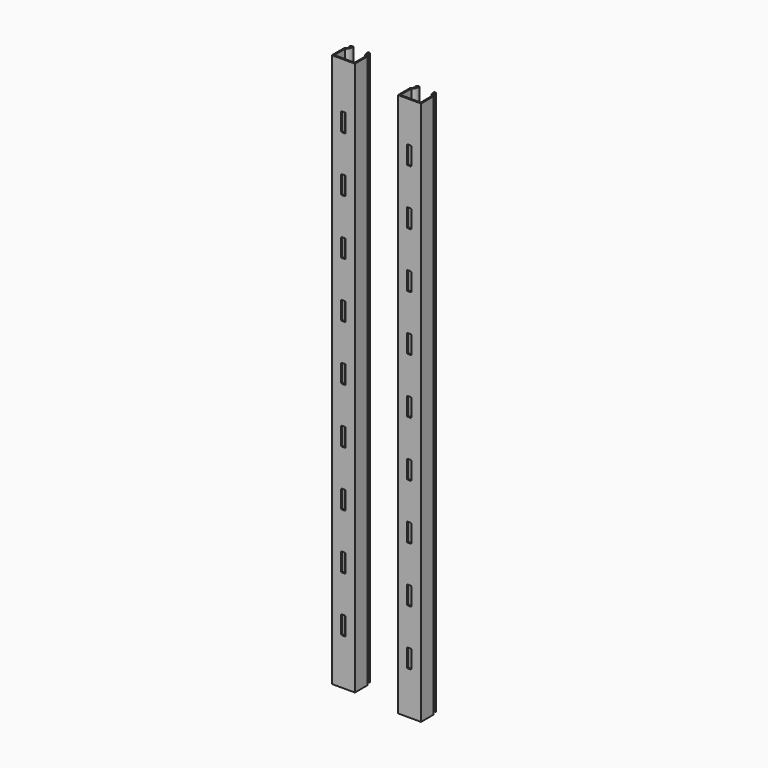
from build123d import *

# Parameters (mm, degrees)
F1_DEPTH = 300
F3_DEPTH = 25
F5_DEPTH = 295
F7_DEPTH = 25


# Not quite as in the source:
# - a feature names something its author has since deleted; it is built from what else it names


with BuildPart() as f1:
    # F0 (on Top) → F1 (new body, symmetric)
    with BuildSketch(Plane.XY):
        with BuildLine():
            Line((-95.8714708686, 0), (-70.8714708686, 0))
            Line((-70.8714708686, 0), (-70.8714708686, 17))
            ThreePointArc((-70.8714708686, 17), (-73.0196975842, 19.1110639706), (-73.8714708686, 22))
            Line((-73.8714708686, 22), (-72.3714708686, 22))
            ThreePointArc((-72.3714708686, 22), (-73.4661714465, 23.4241895875), (-75.2608686682, 23.5))
            ThreePointArc((-75.2608686682, 23.5), (-74.8489206928, 19.4392699226), (-72.3714708686, 16.1955880232))
            Line((-72.3714708686, 16.1955880232), (-72.3714708686, 1.5))
            Line((-72.3714708686, 1.5), (-83.3714708686, 1.5))
            Line((-83.3714708686, 1.5), (-94.3714708686, 1.5))
            Line((-94.3714708686, 1.5), (-94.3714708686, 16.1955880232))
            ThreePointArc((-94.3714708686, 16.1955880232), (-91.8940210443, 19.4392699226), (-91.482073069, 23.5))
            ThreePointArc((-91.482073069, 23.5), (-93.2767702907, 23.4241895875), (-94.3714708686, 22))
            Line((-94.3714708686, 22), (-92.8714708686, 22))
            ThreePointArc((-92.8714708686, 22), (-93.723244153, 19.1110639706), (-95.8714708686, 17))
            Line((-95.8714708686, 17), (-95.8714708686, 0))
        make_face()
    extrude(amount=F1_DEPTH, both=True)

    # F2 (on face) → F3 (cut)
    with BuildSketch(Plane.XZ):
        with BuildLine():
            Line((-84.8714708686, -10), (-83.3714708686, -10))
            Line((-83.3714708686, -10), (-83.3714708686, 0))
            Line((-83.3714708686, 0), (-83.3714708686, 10))
            Line((-83.3714708686, 10), (-84.8714708686, 10))
            ThreePointArc((-84.8714708686, 10), (-85.5785776498, 9.7071067812), (-85.8714708686, 9))
            Line((-85.8714708686, 9), (-85.8714708686, -9))
            ThreePointArc((-85.8714708686, -9), (-85.5785776498, -9.7071067812), (-84.8714708686, -10))
        make_face()
        with BuildLine():
            Line((-83.3714708686, 10), (-83.3714708686, 0))
            Line((-83.3714708686, 0), (-80.8714708686, 0))
            Line((-80.8714708686, 0), (-80.8714708686, 9))
            ThreePointArc((-80.8714708686, 9), (-81.1643640874, 9.7071067812), (-81.8714708686, 10))
            Line((-81.8714708686, 10), (-83.3714708686, 10))
        make_face()
        with BuildLine():
            Line((-83.3714708686, 0), (-83.3714708686, -10))
            Line((-83.3714708686, -10), (-81.8714708686, -10))
            ThreePointArc((-81.8714708686, -10), (-81.1643640874, -9.7071067812), (-80.8714708686, -9))
            Line((-80.8714708686, -9), (-80.8714708686, 0))
            Line((-80.8714708686, 0), (-83.3714708686, 0))
        make_face()
        with BuildLine():
            Line((-81.8714708686, -50), (-83.3714708686, -50))
            Line((-83.3714708686, -50), (-83.3714708686, -60))
            Line((-83.3714708686, -60), (-80.8714708686, -60))
            Line((-80.8714708686, -60), (-80.8714708686, -51))
            ThreePointArc((-80.8714708686, -51), (-81.1643640874, -50.2928932188), (-81.8714708686, -50))
        make_face()
        with BuildLine():
            Line((-80.8714708686, -60), (-83.3714708686, -60))
            Line((-83.3714708686, -60), (-83.3714708686, -70))
            Line((-83.3714708686, -70), (-81.8714708686, -70))
            ThreePointArc((-81.8714708686, -70), (-81.1643640874, -69.7071067812), (-80.8714708686, -69))
            Line((-80.8714708686, -69), (-80.8714708686, -60))
        make_face()
        with BuildLine():
            Line((-83.3714708686, -60), (-83.3714708686, -50))
            Line((-83.3714708686, -50), (-84.8714708686, -50))
            ThreePointArc((-84.8714708686, -50), (-85.5785776498, -50.2928932188), (-85.8714708686, -51))
            Line((-85.8714708686, -51), (-85.8714708686, -60))
            Line((-85.8714708686, -60), (-83.3714708686, -60))
        make_face()
        with BuildLine():
            Line((-83.3714708686, -70), (-83.3714708686, -60))
            Line((-83.3714708686, -60), (-85.8714708686, -60))
            Line((-85.8714708686, -60), (-85.8714708686, -69))
            ThreePointArc((-85.8714708686, -69), (-85.5785776498, -69.7071067812), (-84.8714708686, -70))
            Line((-84.8714708686, -70), (-83.3714708686, -70))
        make_face()
        with BuildLine():
            Line((-81.8714708686, -110), (-83.3714708686, -110))
            Line((-83.3714708686, -110), (-83.3714708686, -120))
            Line((-83.3714708686, -120), (-80.8714708686, -120))
            Line((-80.8714708686, -120), (-80.8714708686, -111))
            ThreePointArc((-80.8714708686, -111), (-81.1643640874, -110.2928932188), (-81.8714708686, -110))
        make_face()
        with BuildLine():
            Line((-80.8714708686, -120), (-83.3714708686, -120))
            Line((-83.3714708686, -120), (-83.3714708686, -130))
            Line((-83.3714708686, -130), (-81.8714708686, -130))
            ThreePointArc((-81.8714708686, -130), (-81.1643640874, -129.7071067812), (-80.8714708686, -129))
            Line((-80.8714708686, -129), (-80.8714708686, -120))
        make_face()
        with BuildLine():
            Line((-83.3714708686, -120), (-83.3714708686, -110))
            Line((-83.3714708686, -110), (-84.8714708686, -110))
            ThreePointArc((-84.8714708686, -110), (-85.5785776498, -110.2928932188), (-85.8714708686, -111))
            Line((-85.8714708686, -111), (-85.8714708686, -129))
            ThreePointArc((-85.8714708686, -129), (-85.5785776498, -129.7071067812), (-84.8714708686, -130))
            Line((-84.8714708686, -130), (-83.3714708686, -130))
            Line((-83.3714708686, -130), (-83.3714708686, -120))
        make_face()
        with BuildLine():
            Line((-83.3714708686, -180), (-83.3714708686, -170))
            Line((-83.3714708686, -170), (-84.8714708686, -170))
            ThreePointArc((-84.8714708686, -170), (-85.5785776498, -170.2928932188), (-85.8714708686, -171))
            Line((-85.8714708686, -171), (-85.8714708686, -180))
            Line((-85.8714708686, -180), (-83.3714708686, -180))
        make_face()
        with BuildLine():
            Line((-83.3714708686, -190), (-83.3714708686, -180))
            Line((-83.3714708686, -180), (-85.8714708686, -180))
            Line((-85.8714708686, -180), (-85.8714708686, -189))
            ThreePointArc((-85.8714708686, -189), (-85.5785776498, -189.7071067812), (-84.8714708686, -190))
            Line((-84.8714708686, -190), (-83.3714708686, -190))
        make_face()
        with BuildLine():
            Line((-80.8714708686, -189), (-80.8714708686, -180))
            Line((-80.8714708686, -180), (-83.3714708686, -180))
            Line((-83.3714708686, -180), (-83.3714708686, -190))
            Line((-83.3714708686, -190), (-81.8714708686, -190))
            ThreePointArc((-81.8714708686, -190), (-81.1643640874, -189.7071067812), (-80.8714708686, -189))
        make_face()
        with BuildLine():
            Line((-81.8714708686, -170), (-83.3714708686, -170))
            Line((-83.3714708686, -170), (-83.3714708686, -180))
            Line((-83.3714708686, -180), (-80.8714708686, -180))
            Line((-80.8714708686, -180), (-80.8714708686, -171))
            ThreePointArc((-80.8714708686, -171), (-81.1643640874, -170.2928932188), (-81.8714708686, -170))
        make_face()
        with BuildLine():
            Line((-83.3714708686, -250), (-83.3714708686, -240))
            Line((-83.3714708686, -240), (-83.3714708686, -230))
            Line((-83.3714708686, -230), (-84.8714708686, -230))
            ThreePointArc((-84.8714708686, -230), (-85.5785776498, -230.2928932188), (-85.8714708686, -231))
            Line((-85.8714708686, -231), (-85.8714708686, -249))
            ThreePointArc((-85.8714708686, -249), (-85.5785776498, -249.7071067812), (-84.8714708686, -250))
            Line((-84.8714708686, -250), (-83.3714708686, -250))
        make_face()
        with BuildLine():
            Line((-83.3714708686, -240), (-80.8714708686, -240))
            Line((-80.8714708686, -240), (-80.8714708686, -231))
            ThreePointArc((-80.8714708686, -231), (-81.1643640874, -230.2928932188), (-81.8714708686, -230))
            Line((-81.8714708686, -230), (-83.3714708686, -230))
            Line((-83.3714708686, -230), (-83.3714708686, -240))
        make_face()
        with BuildLine():
            Line((-80.8714708686, -249), (-80.8714708686, -240))
            Line((-80.8714708686, -240), (-83.3714708686, -240))
            Line((-83.3714708686, -240), (-83.3714708686, -250))
            Line((-83.3714708686, -250), (-81.8714708686, -250))
            ThreePointArc((-81.8714708686, -250), (-81.1643640874, -249.7071067812), (-80.8714708686, -249))
        make_face()
        with BuildLine():
            Line((-83.3714708686, 70), (-83.3714708686, 50))
            Line((-83.3714708686, 50), (-81.8714708686, 50))
            ThreePointArc((-81.8714708686, 50), (-81.1643640874, 50.2928932188), (-80.8714708686, 51))
            Line((-80.8714708686, 51), (-80.8714708686, 69))
            ThreePointArc((-80.8714708686, 69), (-81.1643640874, 69.7071067812), (-81.8714708686, 70))
            Line((-81.8714708686, 70), (-83.3714708686, 70))
        make_face()
        with BuildLine():
            Line((-84.8714708686, 50), (-83.3714708686, 50))
            Line((-83.3714708686, 50), (-83.3714708686, 70))
            Line((-83.3714708686, 70), (-84.8714708686, 70))
            ThreePointArc((-84.8714708686, 70), (-85.5785776498, 69.7071067812), (-85.8714708686, 69))
            Line((-85.8714708686, 69), (-85.8714708686, 51))
            ThreePointArc((-85.8714708686, 51), (-85.5785776498, 50.2928932188), (-84.8714708686, 50))
        make_face()
        with BuildLine():
            Line((-83.3714708686, 120), (-80.8714708686, 120))
            Line((-80.8714708686, 120), (-80.8714708686, 129))
            ThreePointArc((-80.8714708686, 129), (-81.1643640874, 129.7071067812), (-81.8714708686, 130))
            Line((-81.8714708686, 130), (-83.3714708686, 130))
            Line((-83.3714708686, 130), (-83.3714708686, 120))
        make_face()
        with BuildLine():
            Line((-83.3714708686, 120), (-83.3714708686, 110))
            Line((-83.3714708686, 110), (-81.8714708686, 110))
            ThreePointArc((-81.8714708686, 110), (-81.1643640874, 110.2928932188), (-80.8714708686, 111))
            Line((-80.8714708686, 111), (-80.8714708686, 120))
            Line((-80.8714708686, 120), (-83.3714708686, 120))
        make_face()
        with BuildLine():
            Line((-84.8714708686, 110), (-83.3714708686, 110))
            Line((-83.3714708686, 110), (-83.3714708686, 120))
            Line((-83.3714708686, 120), (-83.3714708686, 130))
            Line((-83.3714708686, 130), (-84.8714708686, 130))
            ThreePointArc((-84.8714708686, 130), (-85.5785776498, 129.7071067812), (-85.8714708686, 129))
            Line((-85.8714708686, 129), (-85.8714708686, 111))
            ThreePointArc((-85.8714708686, 111), (-85.5785776498, 110.2928932188), (-84.8714708686, 110))
        make_face()
        with BuildLine():
            Line((-83.3714708686, 180), (-80.8714708686, 180))
            Line((-80.8714708686, 180), (-80.8714708686, 189))
            ThreePointArc((-80.8714708686, 189), (-81.1643640874, 189.7071067812), (-81.8714708686, 190))
            Line((-81.8714708686, 190), (-83.3714708686, 190))
            Line((-83.3714708686, 190), (-83.3714708686, 180))
        make_face()
        with BuildLine():
            Line((-80.8714708686, 171), (-80.8714708686, 180))
            Line((-80.8714708686, 180), (-83.3714708686, 180))
            Line((-83.3714708686, 180), (-83.3714708686, 170))
            Line((-83.3714708686, 170), (-81.8714708686, 170))
            ThreePointArc((-81.8714708686, 170), (-81.1643640874, 170.2928932188), (-80.8714708686, 171))
        make_face()
        with BuildLine():
            Line((-83.3714708686, 170), (-83.3714708686, 180))
            Line((-83.3714708686, 180), (-85.8714708686, 180))
            Line((-85.8714708686, 180), (-85.8714708686, 171))
            ThreePointArc((-85.8714708686, 171), (-85.5785776498, 170.2928932188), (-84.8714708686, 170))
            Line((-84.8714708686, 170), (-83.3714708686, 170))
        make_face()
        with BuildLine():
            Line((-85.8714708686, 180), (-83.3714708686, 180))
            Line((-83.3714708686, 180), (-83.3714708686, 190))
            Line((-83.3714708686, 190), (-84.8714708686, 190))
            ThreePointArc((-84.8714708686, 190), (-85.5785776498, 189.7071067812), (-85.8714708686, 189))
            Line((-85.8714708686, 189), (-85.8714708686, 180))
        make_face()
        with BuildLine():
            Line((-83.3714708686, 240), (-80.8714708686, 240))
            Line((-80.8714708686, 240), (-80.8714708686, 249))
            ThreePointArc((-80.8714708686, 249), (-81.1643640874, 249.7071067812), (-81.8714708686, 250))
            Line((-81.8714708686, 250), (-83.3714708686, 250))
            Line((-83.3714708686, 250), (-83.3714708686, 240))
        make_face()
        with BuildLine():
            Line((-80.8714708686, 231), (-80.8714708686, 240))
            Line((-80.8714708686, 240), (-83.3714708686, 240))
            Line((-83.3714708686, 240), (-83.3714708686, 230))
            Line((-83.3714708686, 230), (-81.8714708686, 230))
            ThreePointArc((-81.8714708686, 230), (-81.1643640874, 230.2928932188), (-80.8714708686, 231))
        make_face()
        with BuildLine():
            Line((-83.3714708686, 230), (-83.3714708686, 240))
            Line((-83.3714708686, 240), (-83.3714708686, 250))
            Line((-83.3714708686, 250), (-84.8714708686, 250))
            ThreePointArc((-84.8714708686, 250), (-85.5785776498, 249.7071067812), (-85.8714708686, 249))
            Line((-85.8714708686, 249), (-85.8714708686, 231))
            ThreePointArc((-85.8714708686, 231), (-85.5785776498, 230.2928932188), (-84.8714708686, 230))
            Line((-84.8714708686, 230), (-83.3714708686, 230))
        make_face()
    extrude(amount=-F3_DEPTH, mode=Mode.SUBTRACT)


with BuildPart() as f5:
    # F4 (on Top) → F5 (new body, symmetric)
    with BuildSketch(Plane.XY):
        with BuildLine():
            Line((-12.5535714286, -14.5844479377), (12.4464285714, -14.5844479377))
            Line((12.4464285714, -14.5844479377), (12.4464285714, 2.4155520623))
            ThreePointArc((12.4464285714, 2.4155520623), (10.2982018558, 4.526616033), (9.4464285714, 7.4155520623))
            Line((9.4464285714, 7.4155520623), (10.9464285714, 7.4155520623))
            ThreePointArc((10.9464285714, 7.4155520623), (9.8517271565, 8.8397400374), (8.0570307718, 8.9155520623))
            ThreePointArc((8.0570307718, 8.9155520623), (8.4689787472, 4.8548219849), (10.9464285714, 1.6111400855))
            Line((10.9464285714, 1.6111400855), (10.9464285714, -13.0844479377))
            Line((10.9464285714, -13.0844479377), (-11.0535714286, -13.0844479377))
            Line((-11.0535714286, -13.0844479377), (-11.0535714286, 1.6111400855))
            ThreePointArc((-11.0535714286, 1.6111400855), (-8.5761216043, 4.8548219849), (-8.164173629, 8.9155520623))
            ThreePointArc((-8.164173629, 8.9155520623), (-9.9588700136, 8.8397400374), (-11.0535714286, 7.4155520623))
            Line((-11.0535714286, 7.4155520623), (-9.5535714286, 7.4155520623))
            ThreePointArc((-9.5535714286, 7.4155520623), (-10.4053447129, 4.526616033), (-12.5535714286, 2.4155520623))
            Line((-12.5535714286, 2.4155520623), (-12.5535714286, -14.5844479377))
        make_face()
    extrude(amount=F5_DEPTH, both=True)

    # F6 (on Front) → F7 (cut)
    with BuildSketch(Plane.XZ):
        with BuildLine():
            Line((-1.974537037, -248.6111111111), (-0.474537037, -248.6111111111))
            Line((-0.474537037, -248.6111111111), (-0.474537037, -238.6111111111))
            Line((-0.474537037, -238.6111111111), (-0.474537037, -228.6111111111))
            Line((-0.474537037, -228.6111111111), (-1.974537037, -228.6111111111))
            ThreePointArc((-1.974537037, -228.6111111111), (-2.6816438182, -228.9040043299), (-2.974537037, -229.6111111111))
            Line((-2.974537037, -229.6111111111), (-2.974537037, -247.6111111111))
            ThreePointArc((-2.974537037, -247.6111111111), (-2.6816438182, -248.3182178923), (-1.974537037, -248.6111111111))
        make_face()
        with BuildLine():
            Line((-0.474537037, -228.6111111111), (-0.474537037, -238.6111111111))
            Line((-0.474537037, -238.6111111111), (2.025462963, -238.6111111111))
            Line((2.025462963, -238.6111111111), (2.025462963, -229.6111111111))
            ThreePointArc((2.025462963, -229.6111111111), (1.7325697441, -228.9040043299), (1.025462963, -228.6111111111))
            Line((1.025462963, -228.6111111111), (-0.474537037, -228.6111111111))
        make_face()
        with BuildLine():
            Line((-0.474537037, -238.6111111111), (-0.474537037, -248.6111111111))
            Line((-0.474537037, -248.6111111111), (1.025462963, -248.6111111111))
            ThreePointArc((1.025462963, -248.6111111111), (1.7325697441, -248.3182178923), (2.025462963, -247.6111111111))
            Line((2.025462963, -247.6111111111), (2.025462963, -238.6111111111))
            Line((2.025462963, -238.6111111111), (-0.474537037, -238.6111111111))
        make_face()
        with BuildLine():
            Line((-0.474537037, -168.6111111111), (-0.474537037, -178.6111111111))
            Line((-0.474537037, -178.6111111111), (2.025462963, -178.6111111111))
            Line((2.025462963, -178.6111111111), (2.025462963, -169.6111111111))
            ThreePointArc((2.025462963, -169.6111111111), (1.7325697441, -168.9040043299), (1.025462963, -168.6111111111))
            Line((1.025462963, -168.6111111111), (-0.474537037, -168.6111111111))
        make_face()
        with BuildLine():
            Line((-2.974537037, -178.6111111111), (-0.474537037, -178.6111111111))
            Line((-0.474537037, -178.6111111111), (-0.474537037, -168.6111111111))
            Line((-0.474537037, -168.6111111111), (-1.974537037, -168.6111111111))
            ThreePointArc((-1.974537037, -168.6111111111), (-2.6816438182, -168.9040043299), (-2.974537037, -169.6111111111))
            Line((-2.974537037, -169.6111111111), (-2.974537037, -178.6111111111))
        make_face()
        with BuildLine():
            Line((-1.974537037, -188.6111111111), (-0.474537037, -188.6111111111))
            Line((-0.474537037, -188.6111111111), (-0.474537037, -178.6111111111))
            Line((-0.474537037, -178.6111111111), (-2.974537037, -178.6111111111))
            Line((-2.974537037, -178.6111111111), (-2.974537037, -187.6111111111))
            ThreePointArc((-2.974537037, -187.6111111111), (-2.6816438182, -188.3182178923), (-1.974537037, -188.6111111111))
        make_face()
        with BuildLine():
            Line((-0.474537037, -178.6111111111), (-0.474537037, -188.6111111111))
            Line((-0.474537037, -188.6111111111), (1.025462963, -188.6111111111))
            ThreePointArc((1.025462963, -188.6111111111), (1.7325697441, -188.3182178923), (2.025462963, -187.6111111111))
            Line((2.025462963, -187.6111111111), (2.025462963, -178.6111111111))
            Line((2.025462963, -178.6111111111), (-0.474537037, -178.6111111111))
        make_face()
        with BuildLine():
            Line((-1.974537037, -128.6111111111), (-0.474537037, -128.6111111111))
            Line((-0.474537037, -128.6111111111), (-0.474537037, -118.6111111111))
            Line((-0.474537037, -118.6111111111), (-0.474537037, -108.6111111111))
            Line((-0.474537037, -108.6111111111), (-1.974537037, -108.6111111111))
            ThreePointArc((-1.974537037, -108.6111111111), (-2.6816438182, -108.9040043299), (-2.974537037, -109.6111111111))
            Line((-2.974537037, -109.6111111111), (-2.974537037, -127.6111111111))
            ThreePointArc((-2.974537037, -127.6111111111), (-2.6816438182, -128.3182178923), (-1.974537037, -128.6111111111))
        make_face()
        with BuildLine():
            Line((-0.474537037, -108.6111111111), (-0.474537037, -118.6111111111))
            Line((-0.474537037, -118.6111111111), (2.025462963, -118.6111111111))
            Line((2.025462963, -118.6111111111), (2.025462963, -109.6111111111))
            ThreePointArc((2.025462963, -109.6111111111), (1.7325697441, -108.9040043299), (1.025462963, -108.6111111111))
            Line((1.025462963, -108.6111111111), (-0.474537037, -108.6111111111))
        make_face()
        with BuildLine():
            Line((-0.474537037, -118.6111111111), (-0.474537037, -128.6111111111))
            Line((-0.474537037, -128.6111111111), (1.025462963, -128.6111111111))
            ThreePointArc((1.025462963, -128.6111111111), (1.7325697441, -128.3182178923), (2.025462963, -127.6111111111))
            Line((2.025462963, -127.6111111111), (2.025462963, -118.6111111111))
            Line((2.025462963, -118.6111111111), (-0.474537037, -118.6111111111))
        make_face()
        with BuildLine():
            Line((-2.974537037, -58.6111111111), (-0.474537037, -58.6111111111))
            Line((-0.474537037, -58.6111111111), (-0.474537037, -48.6111111111))
            Line((-0.474537037, -48.6111111111), (-1.974537037, -48.6111111111))
            ThreePointArc((-1.974537037, -48.6111111111), (-2.6816438182, -48.9040043299), (-2.974537037, -49.6111111111))
            Line((-2.974537037, -49.6111111111), (-2.974537037, -58.6111111111))
        make_face()
        with BuildLine():
            Line((-0.474537037, -48.6111111111), (-0.474537037, -58.6111111111))
            Line((-0.474537037, -58.6111111111), (2.025462963, -58.6111111111))
            Line((2.025462963, -58.6111111111), (2.025462963, -49.6111111111))
            ThreePointArc((2.025462963, -49.6111111111), (1.7325697441, -48.9040043299), (1.025462963, -48.6111111111))
            Line((1.025462963, -48.6111111111), (-0.474537037, -48.6111111111))
        make_face()
        with BuildLine():
            Line((-0.474537037, -58.6111111111), (-0.474537037, -68.6111111111))
            Line((-0.474537037, -68.6111111111), (1.025462963, -68.6111111111))
            ThreePointArc((1.025462963, -68.6111111111), (1.7325697441, -68.3182178923), (2.025462963, -67.6111111111))
            Line((2.025462963, -67.6111111111), (2.025462963, -58.6111111111))
            Line((2.025462963, -58.6111111111), (-0.474537037, -58.6111111111))
        make_face()
        with BuildLine():
            Line((-1.974537037, -68.6111111111), (-0.474537037, -68.6111111111))
            Line((-0.474537037, -68.6111111111), (-0.474537037, -58.6111111111))
            Line((-0.474537037, -58.6111111111), (-2.974537037, -58.6111111111))
            Line((-2.974537037, -58.6111111111), (-2.974537037, -67.6111111111))
            ThreePointArc((-2.974537037, -67.6111111111), (-2.6816438182, -68.3182178923), (-1.974537037, -68.6111111111))
        make_face()
        with BuildLine():
            Line((-1.974537037, -8.6111111111), (-0.474537037, -8.6111111111))
            Line((-0.474537037, -8.6111111111), (-0.474537037, 1.3888888889))
            Line((-0.474537037, 1.3888888889), (-0.474537037, 11.3888888889))
            Line((-0.474537037, 11.3888888889), (-1.974537037, 11.3888888889))
            ThreePointArc((-1.974537037, 11.3888888889), (-2.6816438182, 11.0959956701), (-2.974537037, 10.3888888889))
            Line((-2.974537037, 10.3888888889), (-2.974537037, -7.6111111111))
            ThreePointArc((-2.974537037, -7.6111111111), (-2.6816438182, -8.3182178923), (-1.974537037, -8.6111111111))
        make_face()
        with BuildLine():
            Line((-0.474537037, 11.3888888889), (-0.474537037, 1.3888888889))
            Line((-0.474537037, 1.3888888889), (2.025462963, 1.3888888889))
            Line((2.025462963, 1.3888888889), (2.025462963, 10.3888888889))
            ThreePointArc((2.025462963, 10.3888888889), (1.7325697441, 11.0959956701), (1.025462963, 11.3888888889))
            Line((1.025462963, 11.3888888889), (-0.474537037, 11.3888888889))
        make_face()
        with BuildLine():
            Line((-0.474537037, 1.3888888889), (-0.474537037, -8.6111111111))
            Line((-0.474537037, -8.6111111111), (1.025462963, -8.6111111111))
            ThreePointArc((1.025462963, -8.6111111111), (1.7325697441, -8.3182178923), (2.025462963, -7.6111111111))
            Line((2.025462963, -7.6111111111), (2.025462963, 1.3888888889))
            Line((2.025462963, 1.3888888889), (-0.474537037, 1.3888888889))
        make_face()
        with BuildLine():
            Line((-1.974537037, 51.3888888889), (-0.474537037, 51.3888888889))
            Line((-0.474537037, 51.3888888889), (-0.474537037, 71.3888888889))
            Line((-0.474537037, 71.3888888889), (-1.974537037, 71.3888888889))
            ThreePointArc((-1.974537037, 71.3888888889), (-2.6816438182, 71.0959956701), (-2.974537037, 70.3888888889))
            Line((-2.974537037, 70.3888888889), (-2.974537037, 52.3888888889))
            ThreePointArc((-2.974537037, 52.3888888889), (-2.6816438182, 51.6817821077), (-1.974537037, 51.3888888889))
        make_face()
        with BuildLine():
            Line((-0.474537037, 71.3888888889), (-0.474537037, 51.3888888889))
            Line((-0.474537037, 51.3888888889), (1.025462963, 51.3888888889))
            ThreePointArc((1.025462963, 51.3888888889), (1.7325697441, 51.6817821077), (2.025462963, 52.3888888889))
            Line((2.025462963, 52.3888888889), (2.025462963, 70.3888888889))
            ThreePointArc((2.025462963, 70.3888888889), (1.7325697441, 71.0959956701), (1.025462963, 71.3888888889))
            Line((1.025462963, 71.3888888889), (-0.474537037, 71.3888888889))
        make_face()
        with BuildLine():
            Line((-1.974537037, 111.3888888889), (-0.474537037, 111.3888888889))
            Line((-0.474537037, 111.3888888889), (-0.474537037, 121.3888888889))
            Line((-0.474537037, 121.3888888889), (-0.474537037, 131.3888888889))
            Line((-0.474537037, 131.3888888889), (-1.974537037, 131.3888888889))
            ThreePointArc((-1.974537037, 131.3888888889), (-2.6816438182, 131.0959956701), (-2.974537037, 130.3888888889))
            Line((-2.974537037, 130.3888888889), (-2.974537037, 112.3888888889))
            ThreePointArc((-2.974537037, 112.3888888889), (-2.6816438182, 111.6817821077), (-1.974537037, 111.3888888889))
        make_face()
        with BuildLine():
            Line((-0.474537037, 131.3888888889), (-0.474537037, 121.3888888889))
            Line((-0.474537037, 121.3888888889), (2.025462963, 121.3888888889))
            Line((2.025462963, 121.3888888889), (2.025462963, 130.3888888889))
            ThreePointArc((2.025462963, 130.3888888889), (1.7325697441, 131.0959956701), (1.025462963, 131.3888888889))
            Line((1.025462963, 131.3888888889), (-0.474537037, 131.3888888889))
        make_face()
        with BuildLine():
            Line((-0.474537037, 121.3888888889), (-0.474537037, 111.3888888889))
            Line((-0.474537037, 111.3888888889), (1.025462963, 111.3888888889))
            ThreePointArc((1.025462963, 111.3888888889), (1.7325697441, 111.6817821077), (2.025462963, 112.3888888889))
            Line((2.025462963, 112.3888888889), (2.025462963, 121.3888888889))
            Line((2.025462963, 121.3888888889), (-0.474537037, 121.3888888889))
        make_face()
        with BuildLine():
            Line((-2.974537037, 181.3888888889), (-0.474537037, 181.3888888889))
            Line((-0.474537037, 181.3888888889), (-0.474537037, 191.3888888889))
            Line((-0.474537037, 191.3888888889), (-1.974537037, 191.3888888889))
            ThreePointArc((-1.974537037, 191.3888888889), (-2.6816438182, 191.0959956701), (-2.974537037, 190.3888888889))
            Line((-2.974537037, 190.3888888889), (-2.974537037, 181.3888888889))
        make_face()
        with BuildLine():
            Line((-0.474537037, 191.3888888889), (-0.474537037, 181.3888888889))
            Line((-0.474537037, 181.3888888889), (2.025462963, 181.3888888889))
            Line((2.025462963, 181.3888888889), (2.025462963, 190.3888888889))
            ThreePointArc((2.025462963, 190.3888888889), (1.7325697441, 191.0959956701), (1.025462963, 191.3888888889))
            Line((1.025462963, 191.3888888889), (-0.474537037, 191.3888888889))
        make_face()
        with BuildLine():
            Line((-0.474537037, 181.3888888889), (-0.474537037, 171.3888888889))
            Line((-0.474537037, 171.3888888889), (1.025462963, 171.3888888889))
            ThreePointArc((1.025462963, 171.3888888889), (1.7325697441, 171.6817821077), (2.025462963, 172.3888888889))
            Line((2.025462963, 172.3888888889), (2.025462963, 181.3888888889))
            Line((2.025462963, 181.3888888889), (-0.474537037, 181.3888888889))
        make_face()
        with BuildLine():
            Line((-1.974537037, 171.3888888889), (-0.474537037, 171.3888888889))
            Line((-0.474537037, 171.3888888889), (-0.474537037, 181.3888888889))
            Line((-0.474537037, 181.3888888889), (-2.974537037, 181.3888888889))
            Line((-2.974537037, 181.3888888889), (-2.974537037, 172.3888888889))
            ThreePointArc((-2.974537037, 172.3888888889), (-2.6816438182, 171.6817821077), (-1.974537037, 171.3888888889))
        make_face()
        with BuildLine():
            Line((-1.974537037, 231.3888888889), (-0.474537037, 231.3888888889))
            Line((-0.474537037, 231.3888888889), (-0.474537037, 241.3888888889))
            Line((-0.474537037, 241.3888888889), (-0.474537037, 251.3888888889))
            Line((-0.474537037, 251.3888888889), (-1.974537037, 251.3888888889))
            ThreePointArc((-1.974537037, 251.3888888889), (-2.6816438182, 251.0959956701), (-2.974537037, 250.3888888889))
            Line((-2.974537037, 250.3888888889), (-2.974537037, 232.3888888889))
            ThreePointArc((-2.974537037, 232.3888888889), (-2.6816438182, 231.6817821077), (-1.974537037, 231.3888888889))
        make_face()
        with BuildLine():
            Line((-0.474537037, 251.3888888889), (-0.474537037, 241.3888888889))
            Line((-0.474537037, 241.3888888889), (2.025462963, 241.3888888889))
            Line((2.025462963, 241.3888888889), (2.025462963, 250.3888888889))
            ThreePointArc((2.025462963, 250.3888888889), (1.7325697441, 251.0959956701), (1.025462963, 251.3888888889))
            Line((1.025462963, 251.3888888889), (-0.474537037, 251.3888888889))
        make_face()
        with BuildLine():
            Line((-0.474537037, 241.3888888889), (-0.474537037, 231.3888888889))
            Line((-0.474537037, 231.3888888889), (1.025462963, 231.3888888889))
            ThreePointArc((1.025462963, 231.3888888889), (1.7325697441, 231.6817821077), (2.025462963, 232.3888888889))
            Line((2.025462963, 232.3888888889), (2.025462963, 241.3888888889))
            Line((2.025462963, 241.3888888889), (-0.474537037, 241.3888888889))
        make_face()
    extrude(amount=F7_DEPTH, mode=Mode.SUBTRACT)


solid = Compound([f1.part, f5.part])
